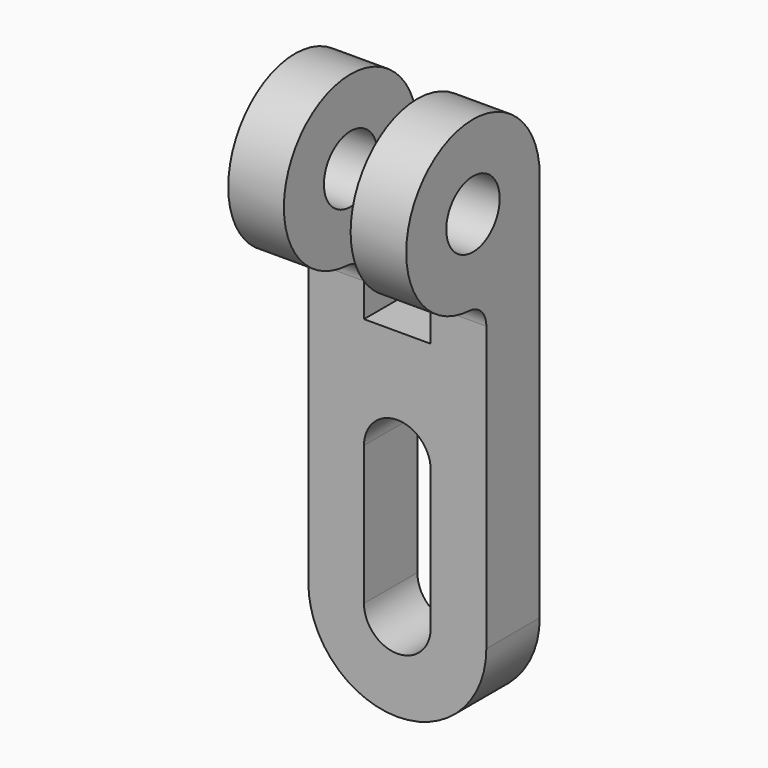
from build123d import *

# Parameters (mm, degrees)
F1_DEPTH = 30
F3_DEPTH = 50
F2_R     = 6
F4_DEPTH = 25.5


# Not quite as in the source:
# - a feature of the source that left no trace in its solid (it failed there, or was rolled back) is left out


with BuildPart() as f1:
    # F0 (on Front) → F1 (new body)
    with BuildSketch(Plane.XZ):
        with BuildLine():
            Line((-16, 85), (-16, 0))
            ThreePointArc((-16, 0), (0, -16), (16, 0))
            Line((16, 0), (16, 85))
            Line((16, 85), (6, 85))
            Line((6, 85), (6, 45))
            Line((6, 45), (-6, 45))
            Line((-6, 45), (-6, 85))
            Line((-6, 85), (-16, 85))
        make_face()
        with BuildLine():
            ThreePointArc((6, 1.3e-09), (-0.0001359155, -5.9999999985), (-5.9999999938, 0.0002718323))
            Line((-5.9999999938, 0.0002718323), (-5.9988673594, 25.0002718323))
            ThreePointArc((-5.9988673594, 25.0002718323), (0.0014044667, 30.9999999938), (6.0011326283, 24.9997281677))
            Line((6.0011326283, 24.9997281677), (6.0000000062, 0))
        make_face(mode=Mode.SUBTRACT)
    extrude(amount=F1_DEPTH)

    # F2 (on Right) → F3 (cut, symmetric)
    with BuildSketch(Plane.YZ):
        with BuildLine():
            ThreePointArc((-15.7894736842, 55.0207900308), (-25.8821437517, 59.6762919758), (-30, 70))
            Line((-30, 70), (-30, -16))
            Line((-30, -16), (-12, -16))
            Line((-12, -16), (-12, 51.026334039))
            ThreePointArc((-12, 51.026334039), (-13.0980949996, 53.7793228454), (-15.7894736842, 55.0207900308))
        make_face()
        with BuildLine():
            Line((-30, 85), (-30, 70))
            ThreePointArc((-30, 70), (-25.6066016991, 80.6066017365), (-14.9999999471, 85))
            Line((-14.9999999471, 85), (-30, 85))
        make_face()
        with BuildLine():
            Line((0, 85), (-14.9999999471, 85))
            ThreePointArc((-14.9999999471, 85), (-4.3933982635, 80.6066016991), (0, 70))
            Line((0, 70), (0, 85))
        make_face()
    extrude(amount=F3_DEPTH, both=True, mode=Mode.SUBTRACT)

    # F2 (on Right) → F4 (cut, symmetric)
    with BuildSketch(Plane.YZ):
        with Locations((-15, 70)):
            Circle(F2_R)
    extrude(amount=F4_DEPTH, both=True, mode=Mode.SUBTRACT)


solid = f1.part
